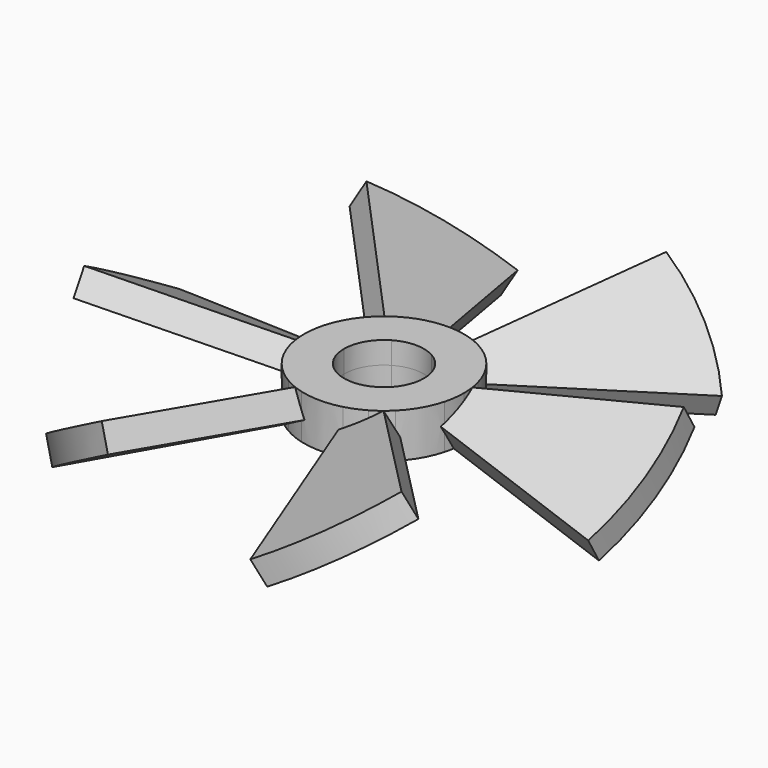
from build123d import *

# Parameters (mm, degrees)
F1_DEPTH      = 5
F1_DEPTH_BACK = 5
F3_ANGLE      = 30
F4_R          = 30
F4_R_2        = 15
F5_DEPTH      = 25
F5_DEPTH_BACK = 25
F0_R          = 15
F6_DEPTH      = 8.306165
F6_DEPTH_BACK = 8.306165
F7_COUNT      = 6


with BuildPart() as f1:
    # F0 (on Top) → F1 (new body, two sides)
    with BuildSketch(Plane.XY) as f1_sk:
        with BuildLine():
            ThreePointArc((28.977775, 7.764571), (29.743346, 3.915786), (30, 0))
            ThreePointArc((30, 0), (29.743346, -3.915786), (28.977775, -7.764571))
            Line((28.977775, -7.764571), (96.592583, -25.881905))
            ThreePointArc((96.592583, -25.881905), (100, 0), (96.592583, 25.881905))
            Line((96.592583, 25.881905), (28.977775, 7.764571))
        make_face()
        with BuildLine():
            ThreePointArc((28.977775, -7.764571), (29.743346, -3.915786), (30, 0))
            ThreePointArc((30, 0), (29.743346, 3.915786), (28.977775, 7.764571))
            Line((28.977775, 7.764571), (22.744913, 6.094481))
            ThreePointArc((22.744913, 6.094481), (23.547266, 0), (22.744913, -6.094481))
            Line((22.744913, -6.094481), (28.977775, -7.764571))
        make_face()
    extrude(amount=F1_DEPTH)
    extrude(f1_sk.sketch, amount=-F1_DEPTH_BACK)


with BuildPart() as f1_1:
    # F3: moved
    add(f1.part.rotate(Axis((-12.394002, 0, 0), (1, 0, 0)), F3_ANGLE))

    # F4 (on Top) → F5 (cut, two sides)
    with BuildSketch(Plane.XY) as f5_sk:
        Circle(F4_R)
        Circle(F4_R_2, mode=Mode.SUBTRACT)
    extrude(amount=-F5_DEPTH, mode=Mode.SUBTRACT)
    extrude(f5_sk.sketch, amount=F5_DEPTH_BACK, mode=Mode.SUBTRACT)

    # F0 (on Top) → F6 (join, two sides)
    with BuildSketch(Plane.XY) as f6_sk:
        with BuildLine():
            Line((22.744913, 6.094481), (28.977775, 7.764571))
            ThreePointArc((28.977775, 7.764571), (-30, 0), (28.977775, -7.764571))
            Line((28.977775, -7.764571), (22.744913, -6.094481))
            ThreePointArc((22.744913, -6.094481), (23.547266, 0), (22.744913, 6.094481))
        make_face()
        Circle(F0_R, mode=Mode.SUBTRACT)
        with BuildLine():
            ThreePointArc((28.977775, -7.764571), (29.743346, -3.915786), (30, 0))
            ThreePointArc((30, 0), (29.743346, 3.915786), (28.977775, 7.764571))
            Line((28.977775, 7.764571), (22.744913, 6.094481))
            ThreePointArc((22.744913, 6.094481), (23.547266, 0), (22.744913, -6.094481))
            Line((22.744913, -6.094481), (28.977775, -7.764571))
        make_face()
    extrude(amount=F6_DEPTH)
    extrude(f6_sk.sketch, amount=-F6_DEPTH_BACK)

    # F7: F1 ×6 about axis
    f7_axis = Axis((0, 0, 0), (0, 0, -1))


with BuildPart() as f1_2:
    add(f1_1.part)
    for i in range(1, F7_COUNT):
        add(f1_1.part.rotate(f7_axis, i * 360 / F7_COUNT))


solid = f1_2.part
